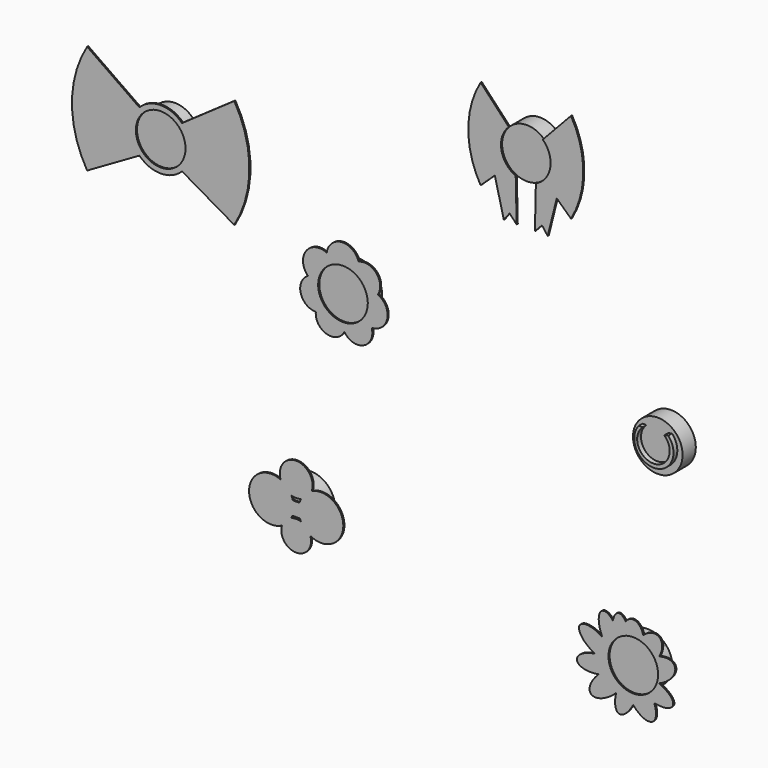
from build123d import *

# Parameters (mm, degrees)
F0_R      = 4.572
F1_DEPTH  = 3.048
F2_R      = 4.572
F3_DEPTH  = 0.254
F4_DEPTH  = 0.254
F5_R      = 4.572
F6_DEPTH  = 0.254
F8_DEPTH  = 0.254
F10_DEPTH = 0.254
F11_DEPTH = 0.254
F12_DEPTH = 0.254
F14_DEPTH = 0.889
F15_R     = 4.572
F16_DEPTH = 0.254
F17_DEPTH = 0.254


# Not quite as in the source:
# - a feature names something its author has since deleted; it is built from what else it names


with BuildPart() as f1:
    # F0 (on Front) → F1 (new body)
    with BuildSketch(Plane.XZ):
        with Locations((-50.1168388258, 43.1532578265)):
            Circle(F0_R)
    extrude(amount=F1_DEPTH)


with BuildPart() as f1b:
    # F0 (on Front) → F1, piece 2 (new body)
    with BuildSketch(Plane.XZ):
        with Locations((-16.5304144873, 28.9974941504)):
            Circle(F0_R)
    extrude(amount=F1_DEPTH)


with BuildPart() as f1c:
    # F0 (on Front) → F1, piece 3 (new body)
    with BuildSketch(Plane.XZ):
        with Locations((17.1497593149, 62.6776661101)):
            Circle(F0_R)
    extrude(amount=F1_DEPTH)


with BuildPart() as f1d:
    # F0 (on Front) → F1, piece 4 (new body)
    with BuildSketch(Plane.XZ):
        with Locations((41.2647664621, 23.0697834727)):
            Circle(F0_R)
    extrude(amount=F1_DEPTH)

    # F13 (on face) → F14 (join)
    with BuildSketch(Plane.XZ.offset(3.048)):
        with BuildLine():
            Line((39.169061929, 25.7497932762), (38.454040885, 25.7497932762))
            ThreePointArc((38.454040885, 25.7497932762), (41.365036345, 19.8476062885), (43.9018234611, 25.9200371802))
            Line((43.9018234611, 25.9200371802), (43.1697778404, 25.7497932762))
            ThreePointArc((43.1697778404, 25.7497932762), (41.1694198847, 20.5202622788), (39.169061929, 25.7497932762))
        make_face()
    extrude(amount=F14_DEPTH)


with BuildPart() as f1e:
    # F0 (on Front) → F1, piece 5 (new body)
    with BuildSketch(Plane.XZ):
        with Locations((-25.1525387743, -8.4548611002)):
            Circle(F0_R)
    extrude(amount=F1_DEPTH)

    # F9 (on face) → F10 (join)
    with BuildSketch(Plane.XZ.offset(3.048)):
        with BuildLine():
            ThreePointArc((-27.7656511155, -12.2065044591), (-27.7627560604, -12.2049370735), (-27.7598622606, -12.2033673713))
            ThreePointArc((-27.7598622606, -12.2033673713), (-27.7607885351, -12.2063058799), (-27.7617114977, -12.2092454305))
            ThreePointArc((-27.7617114977, -12.2092454305), (-25.1525387743, -13.0268611002), (-22.5433660509, -12.2092454305))
            ThreePointArc((-22.5433660509, -12.2092454305), (-22.5442890136, -12.2063058799), (-22.545215288, -12.2033673713))
            ThreePointArc((-22.545215288, -12.2033673713), (-22.5423214883, -12.2049370735), (-22.5394264332, -12.2065044591))
            ThreePointArc((-22.5394264332, -12.2065044591), (-21.0997413686, -10.570993702), (-20.5805387743, -8.4548611002))
            ThreePointArc((-20.5805387743, -8.4548611002), (-27.268671376, -4.4020636945), (-27.7656511155, -12.2065044591))
        make_face()
        with BuildLine():
            ThreePointArc((-26.0518760144, -10.4447166015), (-25.946881329, -10.2205903872), (-25.8555562376, -9.9905552343))
            Line((-25.8555562376, -9.9905552343), (-24.449521311, -9.9905552343))
            ThreePointArc((-24.449521311, -9.9905552343), (-24.3581962196, -10.2205903872), (-24.2532015342, -10.4447166015))
            ThreePointArc((-24.2532015342, -10.4447166015), (-25.1525387743, -10.2925828255), (-26.0518760144, -10.4447166015))
        make_face(mode=Mode.SUBTRACT)
        with BuildLine():
            Line((-24.5450339681, -7.4848332442), (-25.7600435806, -7.4848332442))
            ThreePointArc((-25.7600435806, -7.4848332442), (-25.8792628598, -7.1226518136), (-26.0315071638, -6.7730659198))
            ThreePointArc((-26.0315071638, -6.7730659198), (-25.1525387743, -6.9037664825), (-24.2735703849, -6.7730659198))
            ThreePointArc((-24.2735703849, -6.7730659198), (-24.4258146888, -7.1226518136), (-24.5450339681, -7.4848332442))
        make_face(mode=Mode.SUBTRACT)
    extrude(amount=F10_DEPTH)

    # F9 (on face) → F11 (join)
    with BuildSketch(Plane.XZ.offset(3.048)):
        with BuildLine():
            ThreePointArc((-28.015822622, -4.8459161019), (-33.8335758335, -8.7281953535), (-27.7656511155, -12.2065044591))
            ThreePointArc((-27.7656511155, -12.2065044591), (-27.268671376, -4.4020636945), (-20.5805387743, -8.4548611002))
            ThreePointArc((-20.5805387743, -8.4548611002), (-21.0997413686, -10.570993702), (-22.5394264332, -12.2065044591))
            ThreePointArc((-22.5394264332, -12.2065044591), (-16.4715017151, -8.7281953535), (-22.2892549266, -4.8459161019))
            ThreePointArc((-22.2892549266, -4.8459161019), (-25.1525387743, -0.861955718), (-28.015822622, -4.8459161019))
        make_face()
    extrude(amount=F11_DEPTH)

    # F9 (on face) → F12 (join)
    with BuildSketch(Plane.XZ.offset(3.048)):
        with BuildLine():
            ThreePointArc((-22.5433660509, -12.2092454305), (-25.1525387743, -13.0268611002), (-27.7617114977, -12.2092454305))
            ThreePointArc((-27.7617114977, -12.2092454305), (-25.1525387743, -15.761139375), (-22.5433660509, -12.2092454305))
        make_face()
    extrude(amount=F12_DEPTH)


with BuildPart() as f1f:
    # F0 (on Front) → F1, piece 6 (new body)
    with BuildSketch(Plane.XZ):
        with Locations((36.9537024761, -13.843688319)):
            Circle(F0_R)
    extrude(amount=F1_DEPTH)


with BuildPart() as f3:
    # F2 (on face) → F3 (new body)
    with BuildSketch(Plane.XZ.offset(3.048)):
        with BuildLine():
            ThreePointArc((-46.1906997279, 39.2449638838), (-44.9963244035, 41.0391003561), (-44.577043725, 43.1532578265))
            ThreePointArc((-44.577043725, 43.1532578265), (-44.9963244035, 45.2674152969), (-46.1906997279, 47.0615517692))
            ThreePointArc((-46.1906997279, 47.0615517692), (-50.1168388258, 48.6930529273), (-54.0429779238, 47.0615517692))
            ThreePointArc((-54.0429779238, 47.0615517692), (-55.6566339266, 43.1532578265), (-54.0429779238, 39.2449638838))
            ThreePointArc((-54.0429779238, 39.2449638838), (-50.1168388258, 37.6134627257), (-46.1906997279, 39.2449638838))
        make_face()
        with Locations((-50.1168388258, 43.1532578265)):
            Circle(F2_R, mode=Mode.SUBTRACT)
    extrude(amount=F3_DEPTH)

    # F2 (on face) → F4 (join)
    with BuildSketch(Plane.XZ.offset(3.048)):
        with BuildLine():
            ThreePointArc((-54.0429779238, 39.2449638838), (-55.6566339266, 43.1532578265), (-54.0429779238, 47.0615517692))
            Line((-54.0429779238, 47.0615517692), (-63.6668092272, 53.7716150284))
            ThreePointArc((-63.6668092272, 53.7716150284), (-66.460258801, 43.7272656709), (-63.6668092272, 33.6829163134))
            Line((-63.6668092272, 33.6829163134), (-54.0429779238, 39.2449638838))
        make_face()
        with BuildLine():
            ThreePointArc((-46.1906997279, 47.0615517692), (-44.9963244035, 45.2674152969), (-44.577043725, 43.1532578265))
            ThreePointArc((-44.577043725, 43.1532578265), (-44.9963244035, 41.0391003561), (-46.1906997279, 39.2449638838))
            Line((-46.1906997279, 39.2449638838), (-36.5668684244, 33.6829163134))
            ThreePointArc((-36.5668684244, 33.6829163134), (-33.7734188506, 43.7272656709), (-36.5668684244, 53.7716150284))
            Line((-36.5668684244, 53.7716150284), (-46.1906997279, 47.0615517692))
        make_face()
    extrude(amount=F4_DEPTH)


with BuildPart() as f6:
    # F5 (on face) → F6 (new body)
    with BuildSketch(Plane.XZ.offset(3.048)):
        with BuildLine():
            ThreePointArc((-13.6596207585, 35.1651364151), (-16.7780661139, 37.3241457002), (-19.5250695985, 34.708807408))
            ThreePointArc((-19.5250695985, 34.708807408), (-23.3395170579, 33.7510600732), (-22.996558693, 29.8331947186))
            ThreePointArc((-22.996558693, 29.8331947186), (-24.3186989183, 26.5946300101), (-21.5397571179, 24.4700503772))
            ThreePointArc((-21.5397571179, 24.4700503772), (-19.5358981849, 21.527575028), (-16.2646234139, 22.9319870674))
            ThreePointArc((-16.2646234139, 22.9319870674), (-12.7456705973, 21.8879384489), (-11.2420208719, 25.2363864396))
            ThreePointArc((-11.2420208719, 25.2363864396), (-8.3657556958, 27.6528308307), (-10.0976756394, 30.9863812155))
            ThreePointArc((-10.0976756394, 30.9863812155), (-10.3714504622, 34.3604848558), (-13.6596207585, 35.1651364151))
        make_face()
        with Locations((-16.5304144873, 28.9974941504)):
            Circle(F5_R, mode=Mode.SUBTRACT)
    extrude(amount=F6_DEPTH)


with BuildPart() as f8:
    # F7 (on face) → F8 (new body)
    with BuildSketch(Plane.XZ.offset(3.048)):
        with BuildLine():
            ThreePointArc((15.2929242826, 58.4997063613), (12.6419499117, 61.9142275836), (14.0207789751, 66.0112326736))
            Line((14.0207789751, 66.0112326736), (8.8239936158, 71.547806263))
            ThreePointArc((8.8239936158, 71.547806263), (6.557678528, 63.2053360056), (8.8239936158, 54.8628657482))
            Line((8.8239936158, 54.8628657482), (11.4410703502, 57.3193283668))
            Line((11.4410703502, 57.3193283668), (13.1085459143, 50.6624095142))
            Line((13.1085459143, 50.6624095142), (14.1626789236, 52.0539368398))
            Line((14.1626789236, 52.0539368398), (15.4688060284, 50.6624095142))
            Line((15.4688060284, 50.6624095142), (15.2929242826, 58.4997063613))
        make_face()
    extrude(amount=F8_DEPTH)


with BuildPart() as f8b:
    # F7 (on face) → F8, piece 2 (new body)
    with BuildSketch(Plane.XZ.offset(3.048)):
        with BuildLine():
            Line((25.4755250141, 71.547806263), (20.2787396548, 66.0112326736))
            ThreePointArc((20.2787396548, 66.0112326736), (21.3455239719, 64.4939102961), (21.7217593149, 62.6776661101))
            ThreePointArc((21.7217593149, 62.6776661101), (20.9833368717, 60.1863076221), (19.0065943473, 58.4997063613))
            Line((19.0065943473, 58.4997063613), (18.8307126015, 50.6624095142))
            Line((18.8307126015, 50.6624095142), (20.1368397063, 52.0539368398))
            Line((20.1368397063, 52.0539368398), (21.1909727156, 50.6624095142))
            Line((21.1909727156, 50.6624095142), (22.8584482797, 57.3193283668))
            Line((22.8584482797, 57.3193283668), (25.4755250141, 54.8628657482))
            ThreePointArc((25.4755250141, 54.8628657482), (27.7418401019, 63.2053360056), (25.4755250141, 71.547806263))
        make_face()
    extrude(amount=F8_DEPTH)


with BuildPart() as f16:
    # F15 (on face) → F16 (new body)
    with BuildSketch(Plane.XZ.offset(3.048)):
        with BuildLine():
            add(Edge.make_bspline(
                [(41.6648630143, -15.2390344061), (41.6705784172, -15.2368122218), (41.6762925471, -15.234576702)],
                knots=[1.3218793152, 1.3218793152, 1.3218793152, 1.3254349014, 1.3254349014, 1.3254349014], degree=2, weights=[1, 0.9999984197, 1]))
            ThreePointArc((41.6762925471, -15.234576702), (41.8264561697, -14.5463254332), (41.8768546648, -13.843688319))
            ThreePointArc((41.8768546648, -13.843688319), (32.0815577609, -13.1368408484), (41.6738817208, -15.2427363419))
            add(Edge.make_bspline(
                [(41.6738817208, -15.2427363419), (41.6693741731, -15.2408830764), (41.6648630143, -15.2390344061)],
                knots=[1.403416121, 1.403416121, 1.403416121, 1.4058935999, 1.4058935999, 1.4058935999], degree=2, weights=[1, 0.9999992328, 1]))
        make_face()
        with Locations((36.9537024761, -13.843688319)):
            Circle(F15_R, mode=Mode.SUBTRACT)
    extrude(amount=F16_DEPTH)

    # F15 (on face) → F17 (join)
    with BuildSketch(Plane.XZ.offset(3.048)):
        with BuildLine():
            add(Edge.make_bspline(
                [(41.7560204642, -10.852187672), (42.9442202223, -8.7316533831), (41.7581009403, -7.7370513046), (40.5719816583, -6.742449226), (38.7836838803, -8.3597805514)],
                knots=[1.8004304812, 1.8004304812, 1.8004304812, 3.1154810535, 3.1154810535, 4.4305316258, 4.4305316258, 4.4305316258], degree=2, weights=[1, 0.7915070997, 1, 0.7915070997, 1]))
            add(Edge.make_bspline(
                [(38.7836838803, -8.3597805514), (37.8080650614, -4.2221141352), (35.5526716348, -7.1630860748)],
                knots=[1.8962791896, 1.8962791896, 1.8962791896, 3.8804745915, 3.8804745915, 3.8804745915], degree=2, weights=[1, 0.5469349221, 1]))
            add(Edge.make_bspline(
                [(35.5526716348, -7.1630860748), (33.8212450201, -4.4127673116), (33.208474958, -7.8040858808)],
                knots=[2.3351725788, 2.3351725788, 2.3351725788, 4.0446381263, 4.0446381263, 4.0446381263], degree=2, weights=[1, 0.6564201275, 1]))
            add(Edge.make_bspline(
                [(33.208474958, -7.8040858808), (31.6542458722, -5.8973253477), (30.8559910548, -7.2258627428), (30.0577362374, -8.5544001379), (31.2408004206, -11.0788913032)],
                knots=[2.1423080312, 2.1423080312, 2.1423080312, 3.4784722128, 3.4784722128, 4.8146363945, 4.8146363945, 4.8146363945], degree=2, weights=[1, 0.7850112183, 1, 0.7850112183, 1]))
            add(Edge.make_bspline(
                [(31.2408004206, -11.0788913032), (27.8043891641, -8.8407926999), (27.0308297753, -10.6514127061), (26.2572703865, -12.4620327122), (29.8853455788, -14.2515160422)],
                knots=[4.6590235268, 4.6590235268, 4.6590235268, 6.3540233804, 6.3540233804, 8.049023234, 8.049023234, 8.049023234], degree=2, weights=[1, 0.6618593374, 1, 0.6618593374, 1]))
            add(Edge.make_bspline(
                [(29.8853455788, -14.2515160422), (26.2010922389, -14.7376493192), (26.5712385154, -16.4086617334), (26.9413847919, -18.0796741475), (30.5755640837, -17.3674833325)],
                knots=[4.6771836117, 4.6771836117, 4.6771836117, 6.3156725157, 6.3156725157, 7.9541614196, 7.9541614196, 7.9541614196], degree=2, weights=[1, 0.6827734283, 1, 0.6827734283, 1]))
            add(Edge.make_bspline(
                [(30.5755640837, -17.3674833325), (27.7019361471, -20.1309650501), (29.3189782299, -21.1327909254), (30.9360203128, -22.1346168008), (33.7788079322, -19.352028204)],
                knots=[4.8491447248, 4.8491447248, 4.8491447248, 6.4294772241, 6.4294772241, 8.0098097235, 8.0098097235, 8.0098097235], degree=2, weights=[1, 0.7037272099, 1, 0.7037272099, 1]))
            add(Edge.make_bspline(
                [(33.7788079322, -19.352028204), (31.4798162969, -30.2625741033), (36.9266500341, -20.2799790342)],
                knots=[5.1077160659, 5.1077160659, 5.1077160659, 7.5205710794, 7.5205710794, 7.5205710794], degree=2, weights=[1, 0.3563596232, 1]))
            add(Edge.make_bspline(
                [(36.9266500341, -20.2799790342), (44.6356262609, -29.1657064525), (40.8229500563, -18.6985689053)],
                knots=[4.9478486652, 4.9478486652, 4.9478486652, 7.4042939234, 7.4042939234, 7.4042939234], degree=2, weights=[1, 0.3359123505, 1]))
            add(Edge.make_bspline(
                [(40.8229500563, -18.6985689053), (43.938821437, -19.3485042204), (44.2937268187, -17.9071504359), (44.6486322004, -16.4657966514), (41.6738817208, -15.2427363419)],
                knots=[4.9453056813, 4.9453056813, 4.9453056813, 6.3159535548, 6.3159535548, 7.6866014282, 7.6866014282, 7.6866014282], degree=2, weights=[1, 0.7742140604, 1, 0.7742140604, 1]))
            ThreePointArc((41.6738817208, -15.2427363419), (32.0815577609, -13.1368408484), (41.8768546648, -13.843688319))
            ThreePointArc((41.8768546648, -13.843688319), (41.8264561697, -14.5463254332), (41.6762925471, -15.234576702))
            add(Edge.make_bspline(
                [(41.6762925471, -15.234576702), (44.6527596504, -14.0701034918), (44.6897845291, -12.0349641326), (44.7268094078, -9.9998247735), (41.7560204642, -10.852187672)],
                knots=[1.3254349014, 1.3254349014, 1.3254349014, 2.8194755544, 2.8194755544, 4.3135162075, 4.3135162075, 4.3135162075], degree=2, weights=[1, 0.7337166787, 1, 0.7337166787, 1]))
        make_face()
    extrude(amount=F17_DEPTH)


solid = Compound([f1.part, f1b.part, f1c.part, f1d.part, f1e.part, f1f.part, f3.part, f6.part, f8.part, f8b.part, f16.part])
